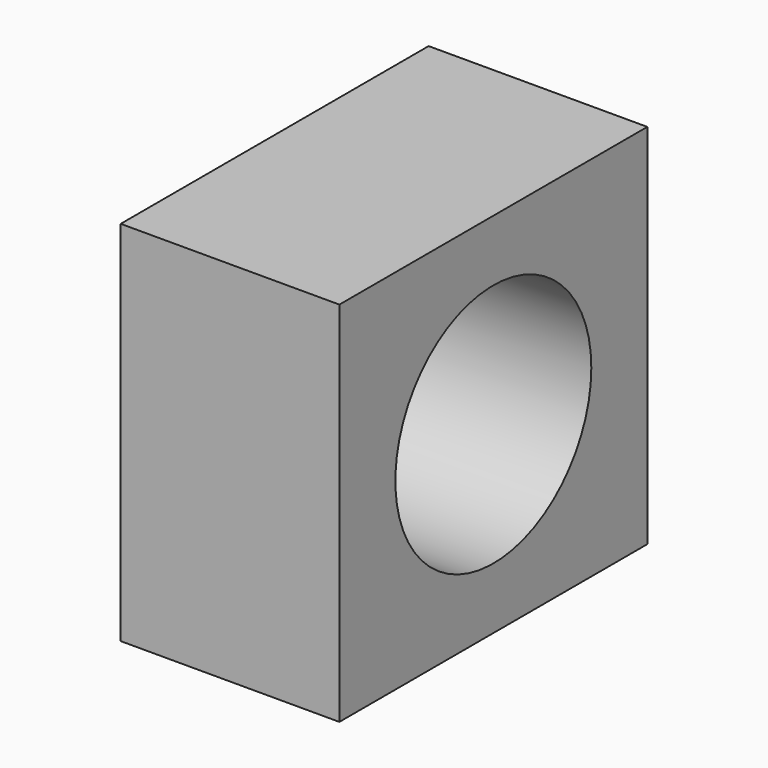
from build123d import *

# Parameters (mm, degrees)
F0_W     = 79.375
F0_H     = 133.35
F1_DEPTH = 139.7
F2_R     = 44.45
F3_DEPTH = 76.2
F4_W     = 6.35
F4_H     = 101.6
F5_DEPTH = 44.45


# Not quite as in the source:
# - a feature names something its author has since deleted; it is built from what else it names


with BuildPart() as f1:
    # F0 (on Front) → F1 (new body)
    with BuildSketch(Plane.XZ):
        Rectangle(F0_W, F0_H)
    extrude(amount=F1_DEPTH)

    # F2 (on face) → F3 (cut)
    with BuildSketch(Plane.YZ.offset(39.6875)):
        with Locations((-69.85, 0)):
            Circle(F2_R)
    extrude(amount=-F3_DEPTH, mode=Mode.SUBTRACT)

    # F4 (on Right) → F5 (join)
    with BuildSketch(Plane.YZ):
        with Locations((-8.2414448261, 0)):
            Rectangle(F4_W, F4_H)
    extrude(amount=-F5_DEPTH)


solid = f1.part
